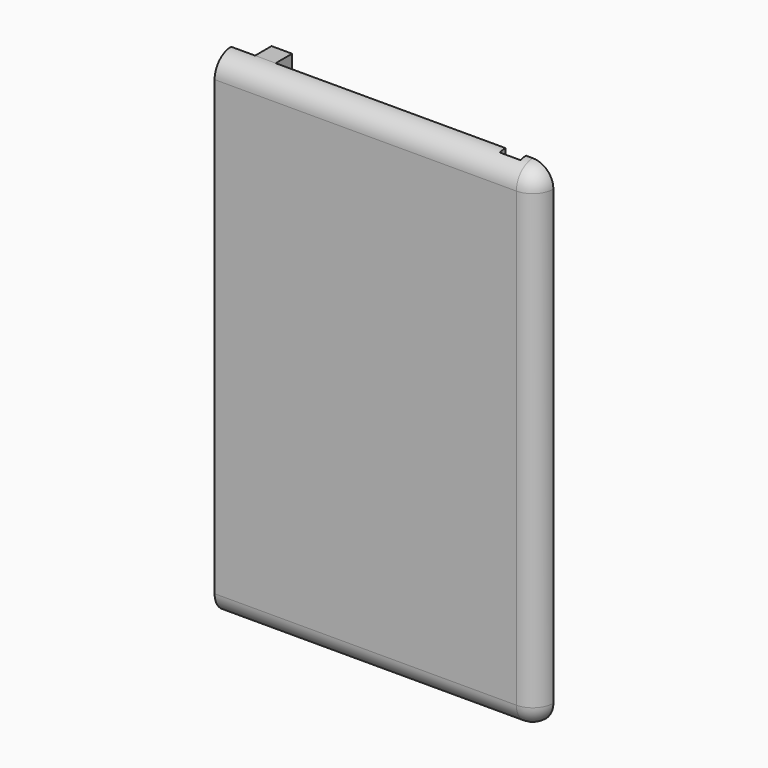
from build123d import *

# Parameters (mm, degrees)
F0_W         = 298.45
F0_H         = 457.2
F1_DEPTH     = 19.05
F3_W         = 19.05
F3_H         = 457.2
F4_DEPTH     = 6.35
F5_T1_DEPTH  = 327.025
F5_T3_DEPTH  = 419.1
F5_T5_DEPTH  = 47.625
F5_S9_W      = 19.05
F5_S9_H      = 19.05
F5_T10_DEPTH = 19.05
F5_S15_W     = 19.05
F5_S15_H     = 19.05
F5_T16_DEPTH = 19.05
F6_W         = 19.05
F6_H         = 457.2
F7_DEPTH     = 19.05
F8_W         = 76.2
F8_H         = 19.05
F9_DEPTH     = 6.35


# Not quite as in the source:
# - a fillet or chamfer that OpenCascade refuses, or shapes differently, is made with other operations: its cross-section is extruded or revolved along the edge and cut away or added


with BuildPart() as f1:
    # F0 (on Front) → F1 (new body)
    with BuildSketch(Plane.XZ):
        Rectangle(F0_W, F0_H)
    extrude(amount=-F1_DEPTH)

    # F3 (on face) → F4 (cut)
    with BuildSketch(Plane(origin=(0, 19.05, 0), x_dir=(-1, 0, 0), z_dir=(0, 1, 0))):
        with Locations((-114.3, 0)):
            Rectangle(F3_W, F3_H)
    extrude(amount=-F4_DEPTH, mode=Mode.SUBTRACT)

    # F5: fillet of radius 19.05 on 5 edges, made by hand

    # F5_s2 → F5_t1 (cut)
    with BuildSketch(Plane.YZ.offset(-196.85)):
        with BuildLine():
            ThreePointArc((19.05, -228.6), (5.5796158184, -223.0203841816), (0, -209.55))
            Line((0, -209.55), (0, -228.6))
            Line((0, -228.6), (19.05, -228.6))
        make_face()
        with BuildLine():
            ThreePointArc((19.05, 228.6), (5.5796158184, 223.0203841816), (0, 209.55))
            Line((0, 209.55), (0, 228.6))
            Line((0, 228.6), (19.05, 228.6))
        make_face()
    extrude(amount=F5_T1_DEPTH, mode=Mode.SUBTRACT)

    # F5_s4 → F5_t3 (cut)
    with BuildSketch(Plane.XY.offset(-209.55)):
        with BuildLine():
            ThreePointArc((130.175, 0), (143.6453841816, 5.5796158184), (149.225, 19.05))
            Line((149.225, 19.05), (149.225, 0))
            Line((149.225, 0), (130.175, 0))
        make_face()
    extrude(amount=F5_T3_DEPTH, mode=Mode.SUBTRACT)

    # F5_s6 → F5_t5 (cut)
    with BuildSketch(Plane.XZ.offset(-66.675)):
        with BuildLine():
            ThreePointArc((130.175, -228.6), (143.6453841816, -223.0203841816), (149.225, -209.55))
            Line((149.225, -209.55), (149.225, -228.6))
            Line((149.225, -228.6), (130.175, -228.6))
        make_face()
        with BuildLine():
            ThreePointArc((130.175, 228.6), (143.6453841816, 223.0203841816), (149.225, 209.55))
            Line((149.225, 209.55), (149.225, 228.6))
            Line((149.225, 228.6), (130.175, 228.6))
        make_face()
    extrude(amount=F5_T5_DEPTH, mode=Mode.SUBTRACT)


with BuildPart() as f5_tool8:
    # F5_s9 → F5_t10 (new body)
    with BuildSketch(Plane.YZ.offset(130.175)):
        with Locations((9.525, -219.075)):
            Rectangle(F5_S9_W, F5_S9_H)
    extrude(amount=F5_T10_DEPTH)

    # F5_s11 → F5_t12 (revolve, cut)
    with BuildSketch(Plane(origin=(130.175, 19.05, -209.55), x_dir=(0, 0.7071067812, 0.7071067812), z_dir=(0, 0.7071067812, -0.7071067812))):
        with BuildLine():
            ThreePointArc((0, -19.05), (19.05, 0), (0, 19.05))
            Line((0, 19.05), (0, -19.05))
        make_face()
    revolve(axis=Axis((130.175, 19.05, -209.55), (1, 0, 0)), mode=Mode.SUBTRACT)


with BuildPart() as f1_1:
    add(f1.part)

    # F5_t7: cut F5_tool8
    add(f5_tool8.part, mode=Mode.SUBTRACT)


with BuildPart() as f5_tool14:
    # F5_s15 → F5_t16 (new body)
    with BuildSketch(Plane.YZ.offset(130.175)):
        with Locations((9.525, 219.075)):
            Rectangle(F5_S15_W, F5_S15_H)
    extrude(amount=F5_T16_DEPTH)

    # F5_s17 → F5_t18 (revolve, cut)
    with BuildSketch(Plane(origin=(130.175, 19.05, 209.55), x_dir=(0, 0.7071067812, -0.7071067812), z_dir=(0, -0.7071067812, -0.7071067812))):
        with BuildLine():
            ThreePointArc((0, -19.05), (19.05, 0), (0, 19.05))
            Line((0, 19.05), (0, -19.05))
        make_face()
    revolve(axis=Axis((130.175, 19.05, 209.55), (1, 0, 0)), mode=Mode.SUBTRACT)


with BuildPart() as f1_2:
    add(f1_1.part)

    # F5_t13: cut F5_tool14
    add(f5_tool14.part, mode=Mode.SUBTRACT)

    # F6 (on face) → F7 (join)
    with BuildSketch(Plane(origin=(0, 19.05, 0), x_dir=(-1, 0, 0), z_dir=(0, 1, 0))):
        with Locations((117.475, 0)):
            Rectangle(F6_W, F6_H)
    extrude(amount=F7_DEPTH)

    # F8 (on face) → F9 (cut, through all)
    with BuildSketch(Plane(origin=(0, 19.05, 0), x_dir=(-1, 0, 0), z_dir=(0, 1, 0))):
        with Locations((-66.675, 104.775)):
            Rectangle(F8_W, F8_H)
        with Locations((-66.675, -104.775)):
            Rectangle(F8_W, F8_H)
    extrude(amount=-F9_DEPTH, mode=Mode.SUBTRACT)


solid = f1_2.part
